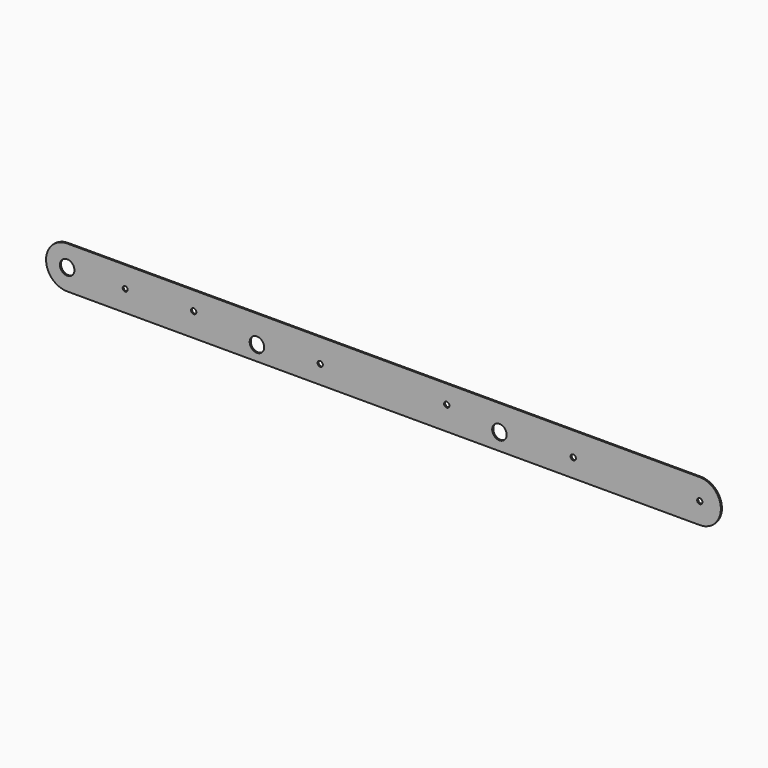
from build123d import *

# Parameters (mm, degrees)
F0_R     = 17.4625
F0_R_2   = 6.35
F1_DEPTH = 3.175


# Not quite as in the source:
# - a feature names something its author has since deleted; it is built from what else it names


with BuildPart() as f1:
    # F0 (on Front) → F1 (new body)
    with BuildSketch(Plane.XZ):
        with BuildLine():
            Line((0, -101.6), (1524, -101.6))
            Line((1524, -101.6), (1524, -57.15))
            ThreePointArc((1524, -57.15), (1517.65, -50.8), (1524, -44.45))
            Line((1524, -44.45), (1524, 0))
            Line((1524, 0), (0, 0))
            ThreePointArc((0, 0), (-35.9210244843, -14.8789755157), (-50.8, -50.8))
            ThreePointArc((-50.8, -50.8), (-35.9210244843, -86.7210244843), (0, -101.6))
        make_face()
        with BuildLine():
            ThreePointArc((17.4625, -50.8), (0, -68.2625), (-17.4625, -50.8))
            ThreePointArc((-17.4625, -50.8), (0, -33.3375), (17.4625, -50.8))
        make_face(mode=Mode.SUBTRACT)
        with BuildLine():
            ThreePointArc((145.7015722418, -50.8), (139.7015722418, -56.8), (133.7015722418, -50.8))
            ThreePointArc((133.7015722418, -50.8), (139.7015722418, -44.8), (145.7015722418, -50.8))
        make_face(mode=Mode.SUBTRACT)
        with Locations((457.2, -65.8510252833)):
            Circle(F0_R, mode=Mode.SUBTRACT)
        with Locations((609.6, -57.15)):
            Circle(F0_R_2, mode=Mode.SUBTRACT)
        with Locations((1041.4, -61.3564662635)):
            Circle(F0_R, mode=Mode.SUBTRACT)
        with Locations((1219.2, -57.15)):
            Circle(F0_R_2, mode=Mode.SUBTRACT)
        with Locations((304.8, -44.45)):
            Circle(F0_R_2, mode=Mode.SUBTRACT)
        with Locations((914.4, -44.45)):
            Circle(F0_R_2, mode=Mode.SUBTRACT)
        with BuildLine():
            Line((1524, -57.15), (1524, -101.6))
            ThreePointArc((1524, -101.6), (1574.8, -50.8), (1524, 0))
            Line((1524, 0), (1524, -44.45))
            ThreePointArc((1524, -44.45), (1528.4901280605, -46.3098719395), (1530.35, -50.8))
            ThreePointArc((1530.35, -50.8), (1528.4901280605, -55.2901280605), (1524, -57.15))
        make_face()
    extrude(amount=F1_DEPTH)


solid = f1.part
